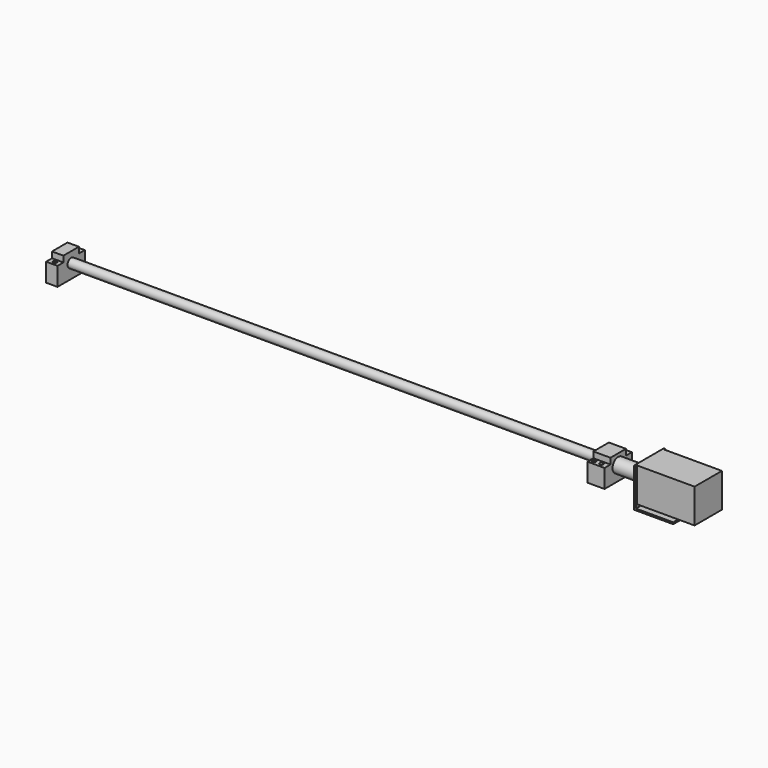
from build123d import *

# Parameters (mm, degrees)
F0_R      = 8
F1_DEPTH  = 980
F3_DEPTH  = 30
F5_DEPTH  = 20
F6_R      = 12.5
F7_DEPTH  = 57
F8_R      = 3.3
F9_DEPTH  = 43.001
F10_W     = 60
F10_H     = 60
F11_DEPTH = 101
F13_DEPTH = 32.5


# Not quite as in the source:
# - a feature names something its author has since deleted; it is built from what else it names


with BuildPart() as f1:
    # F0 (on Right) → F1 (new body)
    with BuildSketch(Plane.YZ):
        Circle(F0_R)
    extrude(amount=F1_DEPTH)

    # F2 (on face) → F3 (join)
    with BuildSketch(Plane.YZ.offset(980)):
        Polygon((30, 7.5), (17, 7.5), (17, 18), (-17, 18), (-17, 7.5), (-30, 7.5), (-30, -25), (30, -25), align=None)
    extrude(amount=-F3_DEPTH)

    # F4 (on face) → F5 (join)
    with BuildSketch(Plane(origin=(0, 0, 0), x_dir=(0, -1, 0), z_dir=(-1, 0, 0))):
        Polygon((17, 7.5), (17, 18), (-17, 18), (-17, 7.5), (-30, 7.5), (-30, -25), (30, -25), (30, 7.5), align=None)
    extrude(amount=-F5_DEPTH)

    # F6 (on face) → F7 (join)
    with BuildSketch(Plane.YZ.offset(980)):
        Circle(F6_R)
    extrude(amount=F7_DEPTH)

    # F8 (on face) → F9 (cut, through all)
    with BuildSketch(Plane.XY.offset(18)):
        with Locations((956, 23)):
            Circle(F8_R)
        with Locations((969, 23)):
            Circle(F8_R)
        with Locations((956, -23)):
            Circle(F8_R)
        with Locations((969, -23)):
            Circle(F8_R)
        with Locations((10, 23)):
            Circle(F8_R)
        with Locations((10, -23)):
            Circle(F8_R)
    extrude(amount=-F9_DEPTH, mode=Mode.SUBTRACT)

    # F10 (on face) → F11 (join)
    with BuildSketch(Plane.YZ.offset(1037)):
        Rectangle(F10_W, F10_H)
    extrude(amount=F11_DEPTH)

    # F12 (on Front) → F13 (join, symmetric)
    with BuildSketch(Plane.XZ):
        Polygon((1037, 30), (1034, 30), (1034, -38.58), (1102.58, -38.58), (1102.58, -35.58), (1037, -35.58), align=None)
    extrude(amount=F13_DEPTH, both=True)


solid = f1.part
